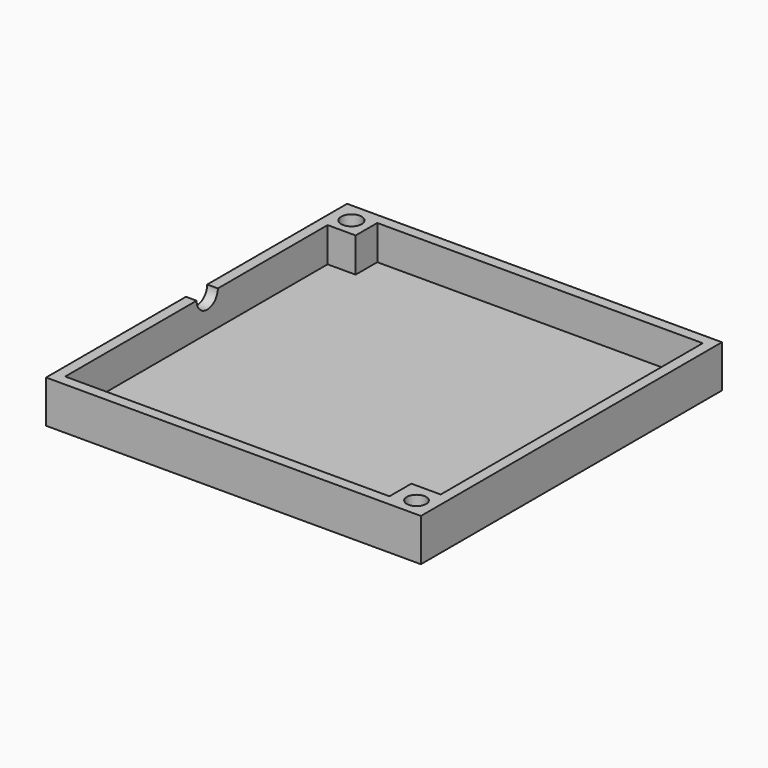
from build123d import *

# Parameters (mm, degrees)
F0_W     = 70.5344155431
F0_H     = 70.8036422729
F0_R     = 1.8180060759
F1_DEPTH = 1.5
F2_DEPTH = 8
F4_D     = 5
F4_DEPTH = 10
F4_TIP   = 1.5021515476


# Not quite as in the source:
# - a feature names something its author has since deleted; it is built from what else it names


with BuildPart() as f1:
    # F0 (on Top) → F1 (new body)
    with BuildSketch(Plane.XY):
        Rectangle(F0_W, F0_H)
        with Locations((31.6813939209, -31.9532230342)):
            Circle(F0_R, mode=Mode.SUBTRACT)
        Polygon((-27.9887095094, 33.4018211365), (33.2672077715, 33.4018211365), (33.2672077715, -28.2499678433), (27.7495980263, -28.2499678433), (27.7495980263, -33.4018211365), (-33.2672077715, -33.4018211365), (-33.2672077715, 28.315147385), (-27.9887095094, 28.315147385), align=None, mode=Mode.SUBTRACT)
        with BuildLine():
            ThreePointArc((-30.620154253, 33.4018211365), (-29.8333233875, 32.6929228695), (-29.5415057982, 31.6748452405))
            ThreePointArc((-29.5415057982, 31.6748452405), (-33.093320688, 30.6567676116), (-30.620154253, 33.4018211365))
        make_face(mode=Mode.SUBTRACT)
        Polygon((33.2672077715, -28.2499678433), (33.2672077715, 33.4018211365), (-27.9887095094, 33.4018211365), (-27.9887095094, 28.315147385), (-33.2672077715, 28.315147385), (-33.2672077715, -33.4018211365), (27.7495980263, -33.4018211365), (27.7495980263, -28.2499678433), align=None)
        with BuildLine():
            ThreePointArc((-30.620154253, 33.4018211365), (-33.093320688, 30.6567676116), (-29.5415057982, 31.6748452405))
            ThreePointArc((-29.5415057982, 31.6748452405), (-29.8333233875, 32.6929228695), (-30.620154253, 33.4018211365))
        make_face()
        with Locations((31.6813939209, -31.9532230342)):
            Circle(F0_R)
    extrude(amount=F1_DEPTH)

    # F0 (on Top) → F2 (join)
    with BuildSketch(Plane.XY):
        Rectangle(F0_W, F0_H)
        with Locations((31.6813939209, -31.9532230342)):
            Circle(F0_R, mode=Mode.SUBTRACT)
        Polygon((-27.9887095094, 33.4018211365), (33.2672077715, 33.4018211365), (33.2672077715, -28.2499678433), (27.7495980263, -28.2499678433), (27.7495980263, -33.4018211365), (-33.2672077715, -33.4018211365), (-33.2672077715, 28.315147385), (-27.9887095094, 28.315147385), align=None, mode=Mode.SUBTRACT)
        with BuildLine():
            ThreePointArc((-30.620154253, 33.4018211365), (-29.8333233875, 32.6929228695), (-29.5415057982, 31.6748452405))
            ThreePointArc((-29.5415057982, 31.6748452405), (-33.093320688, 30.6567676116), (-30.620154253, 33.4018211365))
        make_face(mode=Mode.SUBTRACT)
    extrude(amount=F2_DEPTH)

    # F4
    with Locations(Plane(origin=(-35.2672077715, 0, 0), x_dir=(0, -1, 0), z_dir=(-1, 0, 0))):
        with Locations((0, 8)):
            Hole(F4_D / 2, depth=F4_DEPTH)
            with Locations((0, 0, -(F4_DEPTH + F4_TIP / 2))):  # 118° drill point
                Cone(0, F4_D / 2, F4_TIP, mode=Mode.SUBTRACT)


solid = f1.part
